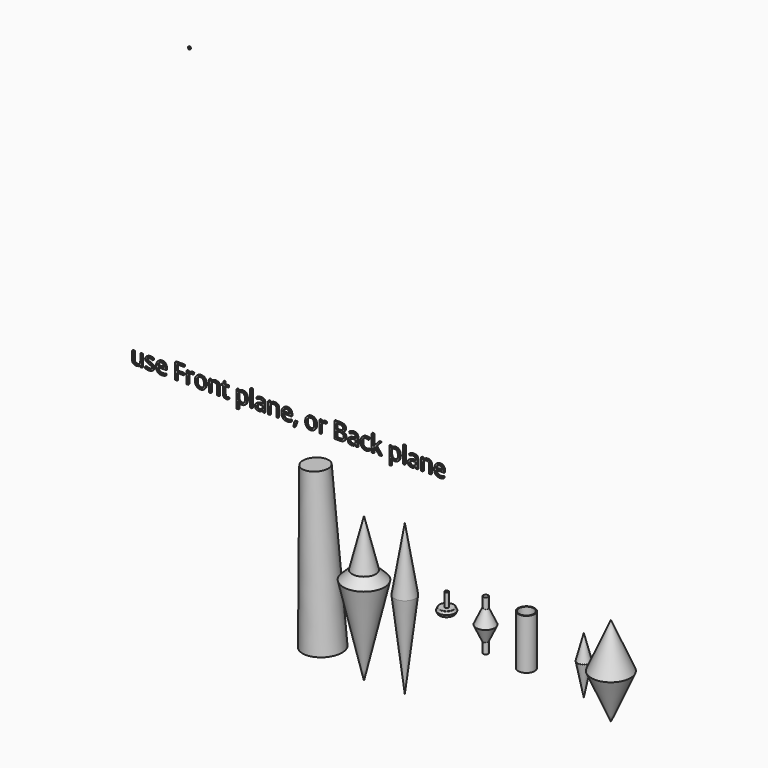
from build123d import *

# Parameters (mm, degrees)
F0_R          = 137.2764362697
F1_DEPTH      = 44.3138945848
F1_TAPER      = 24
F2_R          = 29.677739299
F3_DEPTH      = 266.6965071112
F4_R          = 9.525
F5_R          = 153.8265857183
F6_DEPTH      = 325.889736414
F6_TAPER      = 24.9
F7_R          = 135.1682108016
F8_DEPTH      = 409.1976284981
F7_R_2        = 40.1870084862
F9_T          = -14.2875
F22_TEXT_SIZE = 364.6224737167
F23_DEPTH     = 20.6375
F24_W         = 20.6375
F24_H         = 20.6375
F25_DEPTH     = 25.4
F26_DEPTH     = 12.7


# Not quite as in the source:
# - the program builds the solid bodies; features that only make, move or delete a surface that nothing else refers to are left out
# - Text() gives the source's letters only with a copy of the font that has no kerning and outlines rounded to 1/6400 em; it was checked with that copy


with BuildPart() as f1:
    # F0 (on Top) → F1 (new body, symmetric)
    with BuildSketch(Plane.XY):
        Circle(F0_R)
    extrude(amount=F1_DEPTH, both=True, taper=F1_TAPER)

    # F2 (on Top) → F3 (join)
    with BuildSketch(Plane.XY):
        Circle(F2_R)
    extrude(amount=F3_DEPTH)

    # F4
    f4_edges = [f1.edges().sort_by_distance(p)[0] for p in [
        (-117.546619, 0, -44.313895),
        (-117.546619, 0, 44.313895),
    ]]
    fillet(f4_edges, radius=F4_R)


with BuildPart() as f6:
    # F5 (on Top) → F6 (new body, symmetric)
    with BuildSketch(Plane.XY):
        with Locations((634.1965794563, 0)):
            Circle(F5_R)
    extrude(amount=F6_DEPTH, both=True, taper=F6_TAPER)

    # F7 (on Top) → F8, piece 2 (join, symmetric)
    with BuildSketch(Plane.XY):
        with Locations((638.1026506424, 0)):
            Circle(F7_R_2)
    extrude(amount=F8_DEPTH, both=True)


with BuildPart() as f8:
    # F7 (on Top) → F8 (new body, symmetric)
    with BuildSketch(Plane.XY):
        with Locations((1301.2759685516, 0)):
            Circle(F7_R)
    extrude(amount=F8_DEPTH, both=True)

    # F9
    f9_openings = [f8.faces().sort_by_distance(p)[0] for p in [
        (1301.275969, 0, 409.197628),
    ]]
    offset(amount=F9_T, openings=f9_openings)


with BuildPart() as f11:
    # F10 (on Front) → F11 (revolve)
    with BuildSketch(Plane.XZ):
        Polygon((2343.4345722198, 0), (2238.297700882, 401.4674425125), (2238.297700882, -530.1795005798), align=None)
    revolve(axis=Axis((2238.297700882, 0, -64.3560290337), (0, 0, -1)))


with BuildPart() as f13:
    # F12 (on Front) → F13 (revolve)
    with BuildSketch(Plane.XZ):
        Polygon((-682.4870109558, -1432.4629306793), (-682.4870109558, 1034.4958305359), (-853.4727096558, 0), align=None)
    revolve(axis=Axis((-682.4870109558, 0, -198.9835500717), (0, 0, -1)))


with BuildPart() as f15:
    # F14 (on Front) → F15 (revolve)
    with BuildSketch(Plane.XZ):
        Polygon((-1348.939538002, -1456.3238620758), (-1348.939538002, 916.1272644997), (-1541.4155721664, 140.6374573708), (-1685.0854158401, 0), align=None)
    revolve(axis=Axis((-1348.939538002, 0, -270.0982987881), (0, 0, -1)))


with BuildPart() as f17:
    # F16 (on Front) → F17 (revolve)
    with BuildSketch(Plane.XZ):
        Polygon((-2337.9011154175, -1196.0816383362), (-2020.1072692871, -1226.5272140503), (-2140.7299041748, 1395.4168558121), (-2347.6423839517, 1385.8978394499), align=None)
    revolve(axis=Axis((-2080.418586731, 0, 84.4448208809), (-0.0459564305, 0, 0.9989434451)))


with BuildPart() as f21:
    # F20 (on Front) → F21 (revolve)
    with BuildSketch(Plane.XZ):
        Polygon((2680.6478500366, 734.6506118774), (2680.6478500366, 0), (3000.1239776611, 0), align=None)
        Polygon((3000.1239776611, 0), (2680.6478500366, 0), (2680.6478500366, -734.6506118774), align=None)
    revolve(axis=Axis((2680.6478500366, 0, 367.3253059387), (0, 0, 1)))


with BuildPart() as f23:
    # F22 (on Front) → F23 (new body)
    with BuildSketch(Plane.XZ):
        with Locations((-5146.5322719887, 1879.266500473)):
            Text('use Front plane, or Back plane', F22_TEXT_SIZE, font='Open Sans', text_align=(TextAlign.LEFT, TextAlign.BOTTOM))
    extrude(amount=F23_DEPTH)


with BuildPart() as f25:
    # F24 (on Front) → F25 (new body)
    with BuildSketch(Plane.XZ):
        with Locations((-4193.5299634933, 6726.0655326945)):
            Rectangle(F24_W, F24_H)
    extrude(amount=F25_DEPTH)


with BuildPart() as f26:
    # F24 (on Front) → F26 (new body, symmetric)
    with BuildSketch(Plane.XZ):
        with Locations((-4193.5299634933, 6705.4280326945)):
            Rectangle(F24_W, F24_H)
    extrude(amount=F26_DEPTH, both=True)


solid = Compound([f1.part, f6.part, f8.part, f11.part, f13.part, f15.part, f17.part, f21.part, f23.part, f25.part, f26.part])
